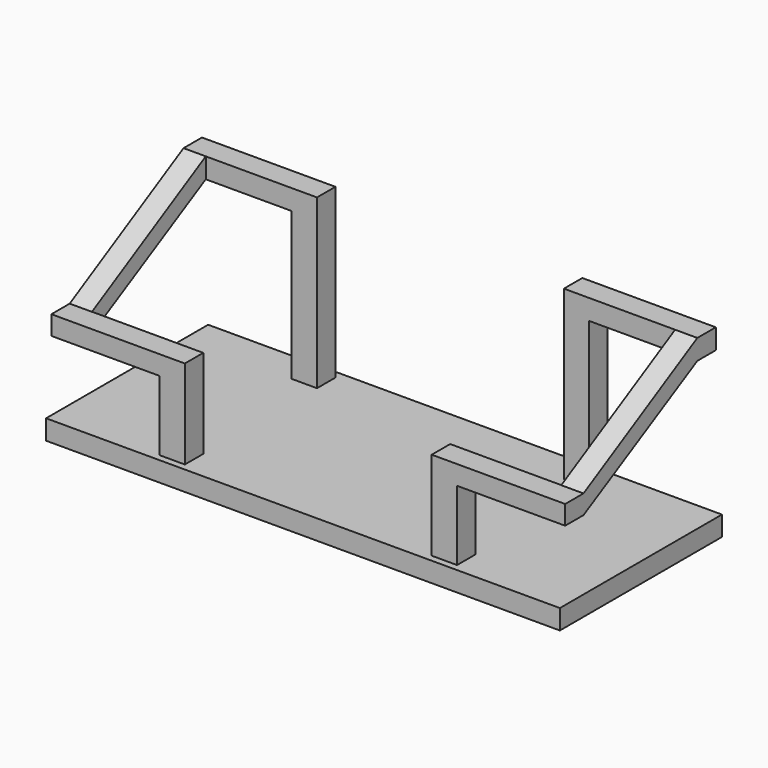
from build123d import *

# Parameters (mm, degrees)
F0_W      = 52
F0_H      = 41
F1_DEPTH  = 4
F2_W      = 5.1310285926
F2_H      = 4.6637309715
F3_DEPTH  = 34
F4_DEPTH  = 18
F5_W      = 4.6637309715
F5_H      = 4.0902358592
F6_DEPTH  = 21.88
F7_W      = 4.6637309715
F7_H      = 3.8742293864
F8_DEPTH  = 21.88
F10_DEPTH = 4.5


with BuildPart() as f1:
    # F0 (on Top) → F1 (new body)
    with BuildSketch(Plane.XY):
        with Locations((-25.150391832, 1.4550268714)):
            Rectangle(F0_W, F0_H)
    extrude(amount=F1_DEPTH)

    # F2 (on face) → F3 (join)
    with BuildSketch(Plane.XY.offset(4)):
        with Locations((-26.7044808716, 18.0663228966)):
            Rectangle(F2_W, F2_H)
    extrude(amount=F3_DEPTH)

    # F2 (on face) → F4 (join)
    with BuildSketch(Plane.XY.offset(4)):
        with Locations((-26.7044808716, -15.3699782677)):
            Rectangle(F2_W, F2_H)
    extrude(amount=F4_DEPTH)

    # F5 (on face) → F6 (join)
    with BuildSketch(Plane(origin=(-29.2699951679, 0, 0), x_dir=(0, -1, 0), z_dir=(-1, 0, 0))):
        with Locations((-18.0663228966, 35.9548820704)):
            Rectangle(F5_W, F5_H)
    extrude(amount=F6_DEPTH)

    # F7 (on face) → F8 (join)
    with BuildSketch(Plane(origin=(-29.2699951679, 0, 0), x_dir=(0, -1, 0), z_dir=(-1, 0, 0))):
        with Locations((15.3699782677, 20.0628853068)):
            Rectangle(F7_W, F7_H)
    extrude(amount=F8_DEPTH)

    # F9 (on face) → F10 (join)
    with BuildSketch(Plane(origin=(-51.1499951679, 0, 0), x_dir=(0, -1, 0), z_dir=(-1, 0, 0))):
        Polygon((14.0116587281, 21.4774478227), (-15.7344574109, 38), (-15.7344574109, 33.9097641408), (13.0349043757, 18.1450489908), (14.0116587281, 18.1450489908), align=None)
    extrude(amount=-F10_DEPTH)

    # F11: F1 across face


with BuildPart() as f1_1:
    add(f1.part)
    add(f1.part.mirror(Plane(origin=(0.849608168, 1.4550268714, 2), x_dir=(0, 1, 0), z_dir=(1, 0, 0))))


solid = f1_1.part
